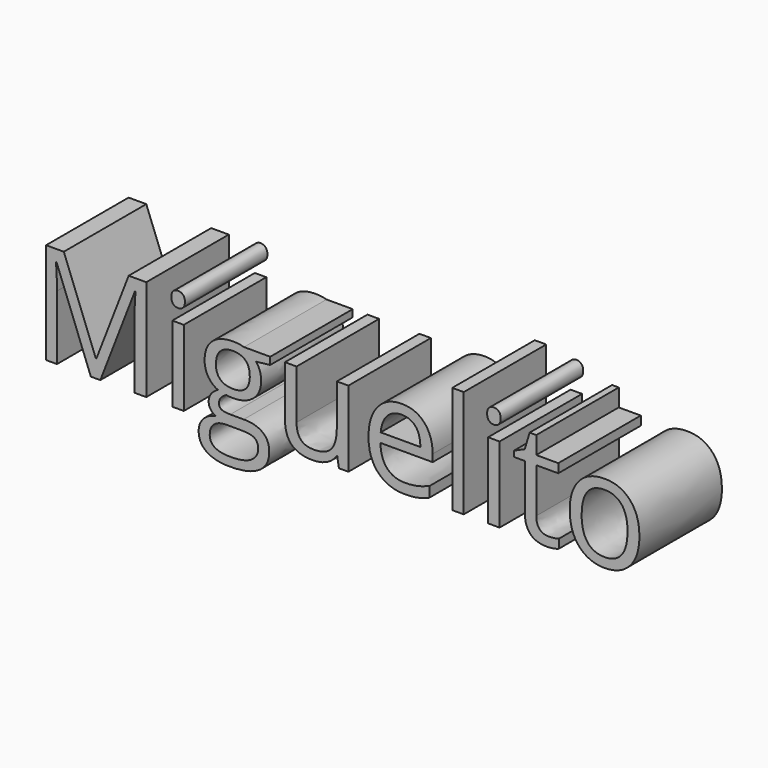
from build123d import *

# Parameters (mm, degrees)
F0_TEXT_SIZE = 34.9014842262
F1_DEPTH     = 25.4


# Not quite as in the source:
# - Text() gives the source's letters only with a copy of the font that has no kerning and outlines rounded to 1/6400 em; it was checked with that copy


with BuildPart() as f1:
    # F0 (on Front) → F1 (new body)
    with BuildSketch(Plane.XZ):
        with Locations((-75.7428066572, 15.290800482)):
            Text('Miguelito', F0_TEXT_SIZE, font='Open Sans', text_align=(TextAlign.LEFT, TextAlign.BOTTOM))
    extrude(amount=F1_DEPTH)


solid = f1.part
